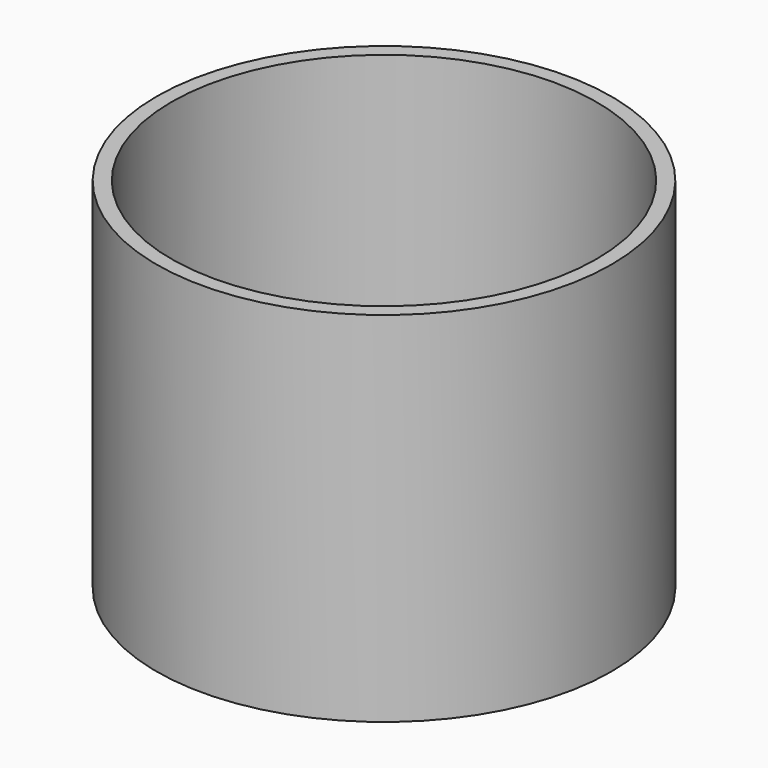
from build123d import *

# Parameters (mm, degrees)
F0_R     = 38.1
F0_R_2   = 35.6
F1_DEPTH = 60


# Not quite as in the source:
# - the program builds the solid bodies; features that only make, move or delete a surface that nothing else refers to are left out


with BuildPart() as f1:
    # F0 (on Top) → F1 (new body)
    with BuildSketch(Plane.XY):
        Circle(F0_R)
        Circle(F0_R_2, mode=Mode.SUBTRACT)
    extrude(amount=F1_DEPTH)


solid = f1.part
